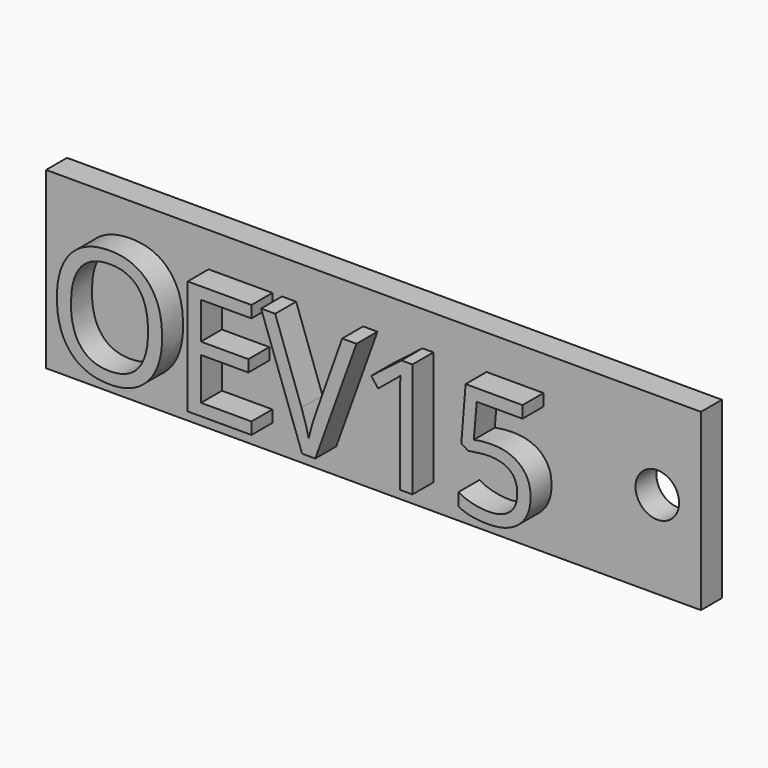
from build123d import *

# Parameters (mm, degrees)
F0_W         = 75
F0_H         = 20
F0_R         = 2.5
F1_DEPTH     = 3
F2_TEXT_SIZE = 18.3603477328
F3_DEPTH     = 3


# Not quite as in the source:
# - Text() gives the source's letters only with a copy of the font that has no kerning and outlines rounded to 1/6400 em; it was checked with that copy


with BuildPart() as f1:
    # F0 (on Front) → F1 (new body)
    with BuildSketch(Plane.XZ):
        with Locations((37.5, -10)):
            Rectangle(F0_W, F0_H)
        with Locations((70, -10)):
            Circle(F0_R, mode=Mode.SUBTRACT)
    extrude(amount=F1_DEPTH)

    # F2 (on face) → F3 (join)
    with BuildSketch(Plane.XZ.offset(3)):
        with Locations((2.5145558175, -17.0760564506)):
            Text('OEV15', F2_TEXT_SIZE, font='Open Sans', text_align=(TextAlign.LEFT, TextAlign.BOTTOM))
    extrude(amount=F3_DEPTH)


solid = f1.part
